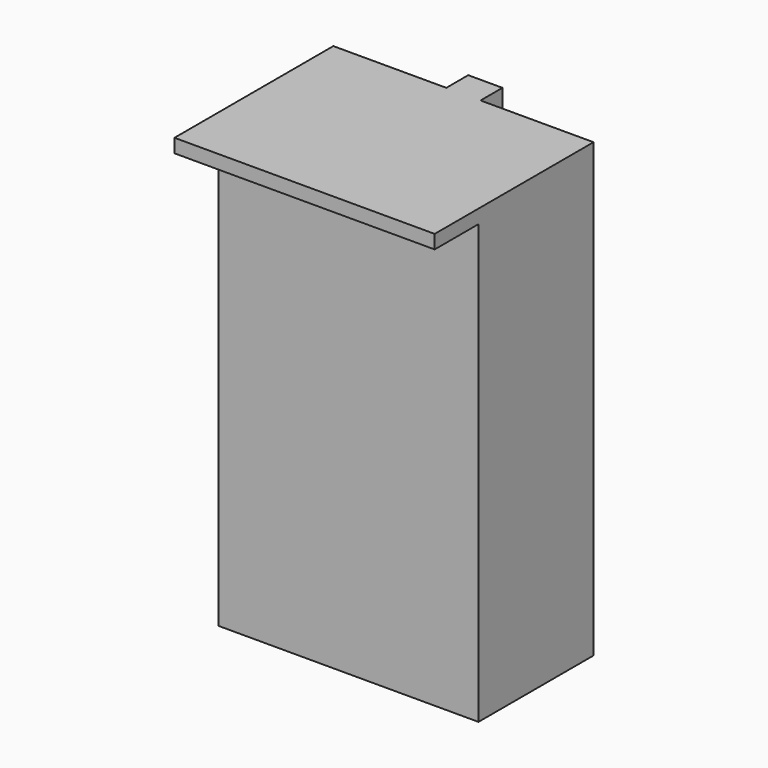
from build123d import *

# Parameters (mm, degrees)
F0_W     = 5
F0_H     = 66
F0_W_2   = 16.5
F1_DEPTH = 21
F2_DEPTH = 4
F3_W     = 38
F3_H     = 2
F4_DEPTH = 8


# Not quite as in the source:
# - a feature names something its author has since deleted; it is built from what else it names


with BuildPart() as f1:
    # F0 (on Front) → F1 (new body)
    with BuildSketch(Plane.XZ):
        with Locations((-35, -33)):
            Rectangle(F0_W, F0_H)
        with Locations((-45.75, -33)):
            Rectangle(F0_W_2, F0_H)
        with Locations((-24.25, -33)):
            Rectangle(F0_W_2, F0_H)
    extrude(amount=F1_DEPTH)

    # F0 (on Front) → F2 (join)
    with BuildSketch(Plane.XZ):
        with Locations((-35, -33)):
            Rectangle(F0_W, F0_H)
    extrude(amount=-F2_DEPTH)

    # F3 (on face) → F4 (join)
    with BuildSketch(Plane.XZ.offset(21)):
        with Locations((-35, -1)):
            Rectangle(F3_W, F3_H)
    extrude(amount=F4_DEPTH)


solid = f1.part
